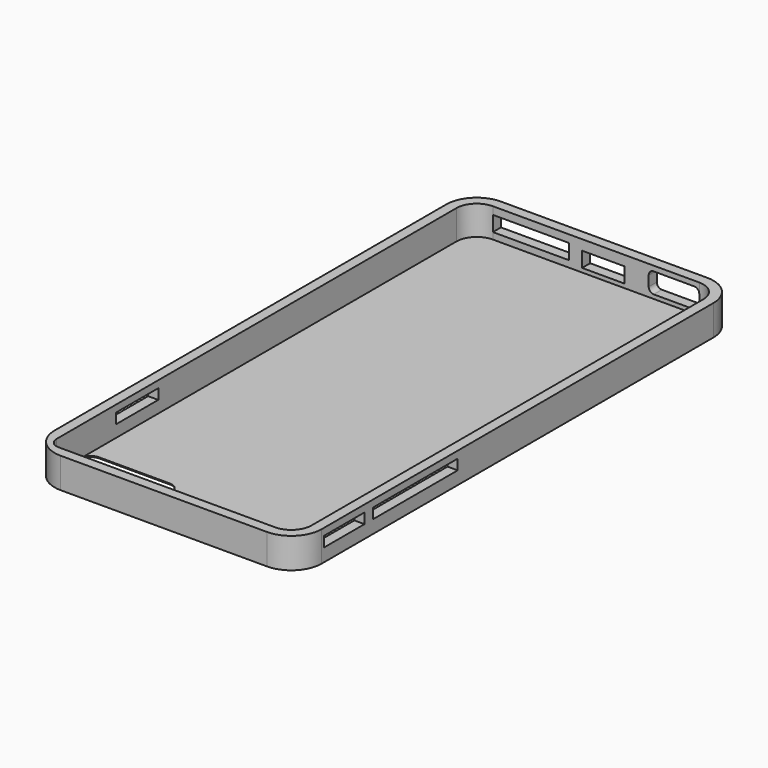
from build123d import *

# Parameters (mm, degrees)
F0_W      = 61.976
F0_H      = 133.096
F1_DEPTH  = 7.62
F2_DEPTH  = 0.254
F3_R      = 7.62
F4_R      = 5.08
F6_DEPTH  = 0.254
F7_W      = 26.6171786934
F7_H      = 2.5910458062
F7_W_2    = 12.6955425367
F8_DEPTH  = 381
F9_W      = 12.6955425367
F9_H      = 2.5910458062
F10_DEPTH = 2.54
F11_W     = 13.3085893467
F11_H     = 2.5910458062
F12_DEPTH = 2.54
F13_W     = 22.86
F13_H     = 12.7
F14_DEPTH = 25.4
F15_R     = 2.54
F16_W     = 12.7
F16_H     = 5.08
F17_DEPTH = 25.4
F18_R     = 1.27
F19_W     = 19.05
F19_H     = 3.81
F20_DEPTH = 25.4
F21_W     = 10.6675168499
F21_H     = 3.81
F22_DEPTH = 25.4


with BuildPart() as f1:
    # F0 (on Top) → F1 (new body)
    with BuildSketch(Plane.XY):
        Polygon((-33.528, 0), (0, 0), (33.528, 0), (33.528, 138.176), (0, 138.176), (-33.528, 138.176), align=None)
        with Locations((0, 69.088)):
            Rectangle(F0_W, F0_H, mode=Mode.SUBTRACT)
    extrude(amount=F1_DEPTH)

    # F0 (on Top) → F2 (join)
    with BuildSketch(Plane.XY):
        with Locations((0, 69.088)):
            Rectangle(F0_W, F0_H)
    extrude(amount=F2_DEPTH)

    # F3
    f3_edges = [f1.edges().sort_by_distance(p)[0] for p in [
        (-33.528, 0, 3.81),
        (33.528, 0, 3.81),
        (33.528, 138.176, 3.81),
        (-33.528, 138.176, 3.81),
    ]]
    fillet(f3_edges, radius=F3_R)

    # F4
    f4_edges = [f1.edges().sort_by_distance(p)[0] for p in [
        (-30.988, 135.636, 3.937),
        (30.988, 135.636, 3.937),
        (-30.988, 2.54, 3.937),
        (30.988, 2.54, 3.937),
    ]]
    fillet(f4_edges, radius=F4_R)

    # F5 (on face) → F6 (join)
    with BuildSketch(Plane.XY):
        Polygon((-30.988, 58.8372340277), (-33.528, 56.507691741), (-30.988, 56.507691741), align=None)
        Polygon((16.764, 69.088), (0, 69.088), (-16.764, 69.088), (-16.764, 61.135802418), (-28.4817721695, 61.135802418), (-30.988, 58.8372340277), (-30.988, 56.507691741), (-16.764, 56.507691741), (-16.764, 52.1295331419), (-26.285154745, 52.1295331419), (-30.988, 46.9043472506), (-30.988, 44.0822318196), (0, 44.0822318196), (30.988, 44.0822318196), (30.988, 47.1902959351), (26.9515123218, 52.1295331419), (0, 52.1295331419), (0, 61.135802418), (24.7533507645, 61.135802418), align=None)
        Polygon((-16.764, 69.088), (0, 69.088), (-16.764, 102.7458906174), align=None)
        Polygon((-30.988, 46.9043472506), (-33.528, 44.0822318196), (-30.988, 44.0822318196), align=None)
    extrude(amount=-F6_DEPTH)

    # F7 (on face) → F8 (cut)
    with BuildSketch(Plane(origin=(-33.528, 0, 0), x_dir=(0, -1, 0), z_dir=(-1, 0, 0))):
        with Locations((-36.9863724336, 4.5639382442)):
            Rectangle(F7_W, F7_H)
        with Locations((-14.7045073099, 4.5639382442)):
            Rectangle(F7_W_2, F7_H)
    extrude(amount=-F8_DEPTH, mode=Mode.SUBTRACT)

    # F9 (on face) → F10 (join)
    with BuildSketch(Plane(origin=(-33.528, 0, 0), x_dir=(0, -1, 0), z_dir=(-1, 0, 0))):
        with Locations((-14.7045073099, 4.5639382442)):
            Rectangle(F9_W, F9_H)
    extrude(amount=-F10_DEPTH)

    # F11 (on face) → F12 (join)
    with BuildSketch(Plane(origin=(-33.528, 0, 0), x_dir=(0, -1, 0), z_dir=(-1, 0, 0))):
        with Locations((-43.640667107, 4.5639382442)):
            Rectangle(F11_W, F11_H)
    extrude(amount=-F12_DEPTH)

    # F13 (on face) → F14 (cut)
    with BuildSketch(Plane.XY):
        with Locations((-19.558, 8.89)):
            Rectangle(F13_W, F13_H)
    extrude(amount=F14_DEPTH, mode=Mode.SUBTRACT)

    # F15
    f15_edges = [f1.edges().sort_by_distance(p)[0] for p in [
        (-8.128, 15.24, 0.127),
        (-8.128, 2.54, 0.127),
        (-30.988, 2.54, 3.81),
        (-30.988, 15.24, 0.127),
    ]]
    fillet(f15_edges, radius=F15_R)

    # F16 (on face) → F17 (cut)
    with BuildSketch(Plane(origin=(0, 138.176, 0), x_dir=(-1, 0, 0), z_dir=(0, 1, 0))):
        with Locations((-19.558, 3.81)):
            Rectangle(F16_W, F16_H)
    extrude(amount=-F17_DEPTH, mode=Mode.SUBTRACT)

    # F18
    f18_edges = [f1.edges().sort_by_distance(p)[0] for p in [
        (13.208, 136.906, 1.27),
        (25.908, 136.906, 1.27),
        (25.908, 136.906, 6.35),
        (13.208, 136.906, 6.35),
    ]]
    fillet(f18_edges, radius=F18_R)

    # F19 (on face) → F20 (cut)
    with BuildSketch(Plane(origin=(0, 138.176, 0), x_dir=(-1, 0, 0), z_dir=(0, 1, 0))):
        with Locations((16.383, 3.81)):
            Rectangle(F19_W, F19_H)
    extrude(amount=-F20_DEPTH, mode=Mode.SUBTRACT)

    # F21 (on face) → F22 (cut)
    with BuildSketch(Plane(origin=(0, 138.176, 0), x_dir=(-1, 0, 0), z_dir=(0, 1, 0))):
        with Locations((-1.8188538961, 3.175)):
            Rectangle(F21_W, F21_H)
    extrude(amount=-F22_DEPTH, mode=Mode.SUBTRACT)


solid = f1.part
